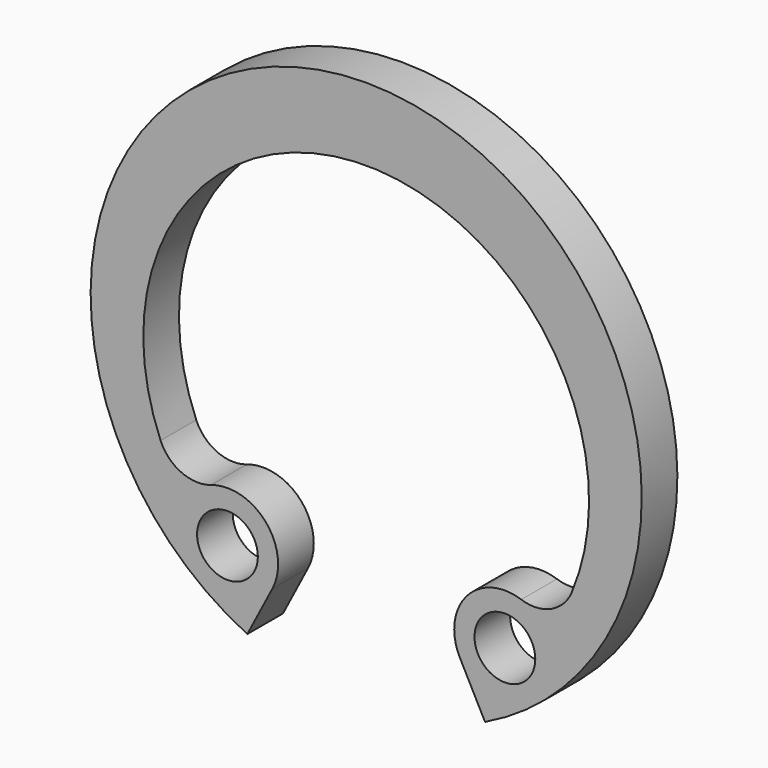
from build123d import *

# Parameters (mm, degrees)
F0_R     = 0.75
F1_DEPTH = 1.1


# Not quite as in the source:
# - a feature of the source that left no trace in its solid (it failed there, or was rolled back) is left out


with BuildPart() as f1:
    # F0 (on Front) → F1 (new body)
    with BuildSketch(Plane.XZ):
        with BuildLine():
            Line((2.3143409039, -4.9458075121), (2.9332922899, -6.1348020622))
            ThreePointArc((2.9332922899, -6.1348020622), (0, 6.8), (-2.9332922899, -6.1348020622))
            Line((-2.9332922899, -6.1348020622), (-2.3143409039, -4.9458075121))
            ThreePointArc((-2.3143409039, -4.9458075121), (-2.4751182669, -3.5538688963), (-3.8270774065, -3.1856991587))
            ThreePointArc((-3.8270774065, -3.1856991587), (-4.5602291476, -3.1514585807), (-5.0725348367, -2.6258857756))
            ThreePointArc((-5.0725348367, -2.6258857756), (0, 5), (5.0725348367, -2.6258857756))
            ThreePointArc((5.0725348367, -2.6258857756), (4.5602291476, -3.1514585807), (3.8270774065, -3.1856991587))
            ThreePointArc((3.8270774065, -3.1856991587), (2.4751182669, -3.5538688963), (2.3143409039, -4.9458075121))
        make_face()
        with Locations((-3.4231044454, -4.3686217456)):
            Circle(F0_R, mode=Mode.SUBTRACT)
        with Locations((3.4231044454, -4.3686217456)):
            Circle(F0_R, mode=Mode.SUBTRACT)
    extrude(amount=F1_DEPTH)


solid = f1.part
